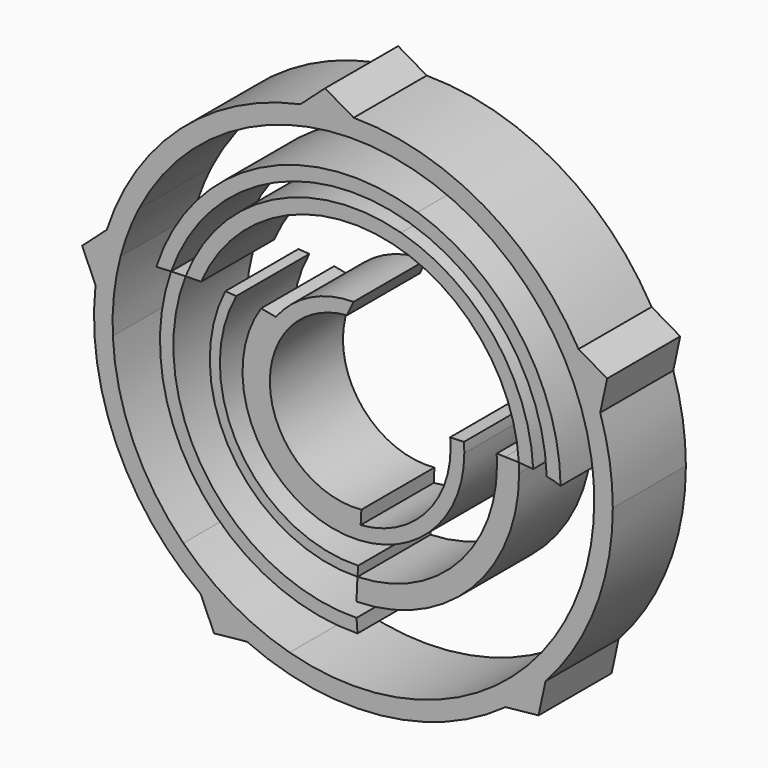
from build123d import *

# Parameters (mm, degrees)
F1_DEPTH = 25.4


with BuildPart() as f1:
    # F0 (on Front) → F1 (new body)
    with BuildSketch(Plane.XZ):
        with BuildLine():
            Line((0.0804563043, 72.1346472531), (-7.8757622136, 76.7543875159))
            Line((-7.8757622136, 76.7543875159), (-14.7280030271, 70.6151523001))
            ThreePointArc((-14.7280030271, 70.6151523001), (-7.3630749336, 71.7579189711), (0.0804563043, 72.1346472531))
        make_face()
        with BuildLine():
            ThreePointArc((62.6077975156, 35.8284453721), (36.2213937543, 62.3812827861), (0.0804563043, 72.1346472531))
            Line((0.0804563043, 72.1346472531), (10.379058307, 66.1548132131))
            ThreePointArc((10.379058307, 66.1548132131), (33.6250311343, 57.9097698478), (52.3091955129, 41.808279412))
            Line((52.3091955129, 41.808279412), (62.6077975156, 35.8284453721))
        make_face()
        with BuildLine():
            Line((10.379058307, 66.1548132131), (0.0804563043, 72.1346472531))
            ThreePointArc((0.0804563043, 72.1346472531), (-7.3630749336, 71.7579189711), (-14.7280030271, 70.6151523001))
            Line((-14.7280030271, 70.6151523001), (-23.5976061943, 62.6684700986))
            ThreePointArc((-23.5976061943, 62.6684700986), (-6.8352870562, 66.6142853558), (10.379058307, 66.1548132131))
        make_face()
        with BuildLine():
            Line((-23.5976061943, 62.6684700986), (-14.7280030271, 70.6151523001))
            ThreePointArc((-14.7280030271, 70.6151523001), (-48.1350992585, 53.7254690711), (-68.5792639553, 22.3673503769))
            Line((-68.5792639553, 22.3673503769), (-59.7096607881, 30.3140325785))
            ThreePointArc((-59.7096607881, 30.3140325785), (-44.684757914, 49.8744079942), (-23.5976061943, 62.6684700986))
        make_face()
        with BuildLine():
            ThreePointArc((68.628988686, 22.214313392), (65.9705211479, 29.1771168386), (62.6077975156, 35.8284453721))
            Line((62.6077975156, 35.8284453721), (52.3091955129, 41.808279412))
            ThreePointArc((52.3091955129, 41.808279412), (61.2417303042, 27.0856905386), (66.1242715931, 10.5718905067))
            Line((66.1242715931, 10.5718905067), (68.628988686, 22.214313392))
        make_face()
        with BuildLine():
            Line((70.5640160335, 31.2087051093), (62.6077975156, 35.8284453721))
            ThreePointArc((62.6077975156, 35.8284453721), (65.9705211479, 29.1771168386), (68.628988686, 22.214313392))
            Line((68.628988686, 22.214313392), (70.5640160335, 31.2087051093))
        make_face()
        with BuildLine():
            ThreePointArc((-70.1811130337, 16.6740871082), (-69.4385618169, 19.5371425839), (-68.5792639553, 22.3673503769))
            Line((-68.5792639553, 22.3673503769), (-75.4315047689, 16.2281151612))
            add(Edge.make_bspline(
                [(-75.4315047689, 16.2281151612), (-73.6801810781, 16.3779407802), (-71.9288512089, 16.5277670762), (-70.1811130337, 16.6740871082)],
                knots=[0, 0, 0, 0, 0.0110848613, 0.0110848613, 0.0110848613, 0.0110848613], degree=3))
        make_face()
        with BuildLine():
            Line((-59.7096607881, 30.3140325785), (-68.5792639553, 22.3673503769))
            ThreePointArc((-68.5792639553, 22.3673503769), (-69.4385618169, 19.5371425839), (-70.1811130337, 16.6740871082))
            add(Edge.make_bspline(
                [(-70.1811130337, 16.6740871082), (-68.362095804, 16.8263745979), (-66.5469692067, 16.9748639956), (-64.7397895139, 17.1156015464)],
                knots=[0.0110848613, 0.0110848613, 0.0110848613, 0.0110848613, 0.0226218032, 0.0226218032, 0.0226218032, 0.0226218032], degree=3))
            ThreePointArc((-64.7397895139, 17.1156015464), (-62.5736850885, 23.8478111585), (-59.7096607881, 30.3140325785))
        make_face()
        with BuildLine():
            ThreePointArc((72.134692122, 0), (71.2528763526, 11.2446173352), (68.628988686, 22.214313392))
            Line((68.628988686, 22.214313392), (66.1242715931, 10.5718905067))
            ThreePointArc((66.1242715931, 10.5718905067), (66.7537762071, 5.3025960338), (66.9640512708, 0))
            ThreePointArc((66.9640512708, 0), (64.145330939, -19.223961125), (55.9264669455, -36.8295324108))
            Line((55.9264669455, -36.8295324108), (53.4217498526, -48.4719552961))
            ThreePointArc((53.4217498526, -48.4719552961), (67.2940386876, -25.9793411127), (72.134692122, 0))
        make_face()
        with BuildLine():
            add(Edge.make_bspline(
                [(-75.4315047689, 16.2281151612), (-73.6801810781, 16.3779407802), (-71.9288512089, 16.5277670762), (-70.1811130337, 16.6740871082)],
                knots=[0, 0, 0, 0, 0.0110848613, 0.0110848613, 0.0110848613, 0.0110848613], degree=3))
            Line((-75.4315047689, 16.2281151612), (-71.7102039728, 7.8141188702))
            ThreePointArc((-71.7102039728, 7.8141188702), (-71.0838323373, 12.2679496162), (-70.1811130337, 16.6740871082))
        make_face()
        with BuildLine():
            add(Edge.make_bspline(
                [(-70.1811130337, 16.6740871082), (-68.362095804, 16.8263745979), (-66.5469692067, 16.9748639956), (-64.7397895139, 17.1156015464)],
                knots=[0.0110848613, 0.0110848613, 0.0110848613, 0.0110848613, 0.0226218032, 0.0226218032, 0.0226218032, 0.0226218032], degree=3))
            ThreePointArc((-70.1811130337, 16.6740871082), (-71.0838323373, 12.2679496162), (-71.7102039728, 7.8141188702))
            Line((-71.7102039728, 7.8141188702), (-66.8933181941, -3.0770348681))
            ThreePointArc((-66.8933181941, -3.0770348681), (-66.5864430839, 7.1013914157), (-64.7397895139, 17.1156015464))
        make_face()
        with BuildLine():
            Line((-66.8933181941, -3.0770348681), (-71.7102039728, 7.8141188702))
            ThreePointArc((-71.7102039728, 7.8141188702), (-65.9705211479, -29.1771168386), (-42.4647723522, -58.3108644818))
            Line((-42.4647723522, -58.3108644818), (-47.2816581308, -47.4197107436))
            ThreePointArc((-47.2816581308, -47.4197107436), (-61.2417303042, -27.0856905386), (-66.8933181941, -3.0770348681))
        make_face()
        with BuildLine():
            ThreePointArc((42.3345913172, -58.4054465401), (48.1350992585, -53.7254690711), (53.4217498526, -48.4719552961))
            Line((53.4217498526, -48.4719552961), (55.9264669455, -36.8295324108))
            ThreePointArc((55.9264669455, -36.8295324108), (44.684757914, -49.8744079942), (30.4879890188, -59.6210255547))
            Line((30.4879890188, -59.6210255547), (42.3345913172, -58.4054465401))
        make_face()
        with BuildLine():
            Line((51.486722505, -57.4663470135), (53.4217498526, -48.4719552961))
            ThreePointArc((53.4217498526, -48.4719552961), (48.1350992585, -53.7254690711), (42.3345913172, -58.4054465401))
            Line((42.3345913172, -58.4054465401), (51.486722505, -57.4663470135))
        make_face()
        with BuildLine():
            ThreePointArc((-29.5913403683, -65.7857612463), (-36.2213937543, -62.3812827861), (-42.4647723522, -58.3108644818))
            Line((-42.4647723522, -58.3108644818), (-38.7434715561, -66.7248607729))
            Line((-38.7434715561, -66.7248607729), (-29.5913403683, -65.7857612463))
        make_face()
        with BuildLine():
            Line((-47.2816581308, -47.4197107436), (-42.4647723522, -58.3108644818))
            ThreePointArc((-42.4647723522, -58.3108644818), (-36.2213937543, -62.3812827861), (-29.5913403683, -65.7857612463))
            Line((-29.5913403683, -65.7857612463), (-17.7447380699, -64.5701822317))
            ThreePointArc((-17.7447380699, -64.5701822317), (-33.6250311343, -57.9097698478), (-47.2816581308, -47.4197107436))
        make_face()
        with BuildLine():
            ThreePointArc((-29.5913403683, -65.7857612463), (7.3630749336, -71.7579189711), (42.3345913172, -58.4054465401))
            Line((42.3345913172, -58.4054465401), (30.4879890188, -59.6210255547))
            ThreePointArc((30.4879890188, -59.6210255547), (6.8352870562, -66.6142853558), (-17.7447380699, -64.5701822317))
            Line((-17.7447380699, -64.5701822317), (-29.5913403683, -65.7857612463))
        make_face()
    extrude(amount=F1_DEPTH)


with BuildPart() as f1b:
    # F0 (on Front) → F1, piece 2 (new body)
    with BuildSketch(Plane.XZ):
        with BuildLine():
            ThreePointArc((17.8474131482, 54.7811527956), (-26.1415508125, 51.3431999277), (-54.7988191164, 17.7930964463))
            add(Edge.make_bspline(
                [(-54.7988191164, 17.7930964463), (-53.4180734669, 17.8701419739), (-52.0468052053, 17.9379460939), (-50.6869602761, 17.9946120432)],
                knots=[0.0440052643, 0.0440052643, 0.0440052643, 0.0440052643, 0.0530367351, 0.0530367351, 0.0530367351, 0.0530367351], degree=3))
            ThreePointArc((-50.6869602761, 17.9946120432), (-24.2822021716, 47.9932147528), (15.5280586181, 51.4961493722))
            add(Edge.make_bspline(
                [(15.5280586181, 51.4961493722), (16.2953998908, 52.5878890346), (17.0695301608, 53.6834646207), (17.8474131482, 54.7811527956)],
                knots=[0.9806259826, 0.9806259826, 0.9806259826, 0.9806259826, 0.9892751554, 0.9892751554, 0.9892751554, 0.9892751554], degree=3))
        make_face()
        with BuildLine():
            add(Edge.make_bspline(
                [(57.6107607755, 0.7107042783), (56.462742198, 1.1538709295), (55.1691307112, 1.5102558583), (53.7564053874, 1.7952393804)],
                knots=[0.6553417422, 0.6553417422, 0.6553417422, 0.6553417422, 0.6691124751, 0.6691124751, 0.6691124751, 0.6691124751], degree=3))
            ThreePointArc((57.6107607755, 0.7107042783), (46.4153784181, 34.1338176009), (17.8474131482, 54.7811527956))
            add(Edge.make_bspline(
                [(15.5280586181, 51.4961493722), (16.2953998908, 52.5878890346), (17.0695301608, 53.6834646207), (17.8474131482, 54.7811527956)],
                knots=[0.9806259826, 0.9806259826, 0.9806259826, 0.9806259826, 0.9892751554, 0.9892751554, 0.9892751554, 0.9892751554], degree=3))
            ThreePointArc((15.5280586181, 51.4961493722), (42.6336645345, 32.7924481089), (53.7564053874, 1.7952393804))
        make_face()
    extrude(amount=F1_DEPTH)


with BuildPart() as f1c:
    # F0 (on Front) → F1, piece 3 (new body)
    with BuildSketch(Plane.XZ):
        with BuildLine():
            add(Edge.make_bspline(
                [(-50.6869602761, 17.9946120432), (-49.3314822975, 18.0510960178), (-47.9873544002, 18.0965132441), (-46.6565038412, 18.1289851741)],
                knots=[0.0530367351, 0.0530367351, 0.0530367351, 0.0530367351, 0.0620392027, 0.0620392027, 0.0620392027, 0.0620392027], degree=3))
            ThreePointArc((-50.6869602761, 17.9946120432), (-43.604859977, -31.4895250996), (1.141385438, -53.7742619093))
            add(Edge.make_bspline(
                [(0.8706699494, -50.0472915148), (0.9119172038, -51.3735505285), (0.9980162573, -52.6210201223), (1.141385438, -53.7742619093)],
                knots=[0.3429048112, 0.3429048112, 0.3429048112, 0.3429048112, 0.3552562401, 0.3552562401, 0.3552562401, 0.3552562401], degree=3))
            ThreePointArc((0.8706699494, -50.0472915148), (-41.0619875564, -28.6252097293), (-46.6565038412, 18.1289851741))
        make_face()
    extrude(amount=F1_DEPTH)


with BuildPart() as f1d:
    # F0 (on Front) → F1, piece 4 (new body)
    with BuildSketch(Plane.XZ):
        with BuildLine():
            ThreePointArc((13.2700106945, 48.2638194748), (-22.4875863699, 44.7191000959), (-46.6565038412, 18.1289851741))
            add(Edge.make_bspline(
                [(-46.6565038412, 18.1289851741), (-45.202639449, 18.1644585655), (-43.7646203485, 18.1844829268), (-42.3449591404, 18.1866091603)],
                knots=[0.0620392027, 0.0620392027, 0.0620392027, 0.0620392027, 0.0718737908, 0.0718737908, 0.0718737908, 0.0718737908], degree=3))
            ThreePointArc((-42.3449591404, 18.1866091603), (-20.6004330804, 41.2246343132), (10.878347446, 44.782919447))
            add(Edge.make_bspline(
                [(10.878347446, 44.782919447), (11.6616317718, 45.9353294378), (12.4601226636, 47.0963501665), (13.2700106945, 48.2638194748)],
                knots=[0.9627272628, 0.9627272628, 0.9627272628, 0.9627272628, 0.9720558065, 0.9720558065, 0.9720558065, 0.9720558065], degree=3))
        make_face()
        with BuildLine():
            add(Edge.make_bspline(
                [(49.9988649095, 2.3670576439), (48.7257298476, 2.5084241824), (47.3905488256, 2.6123363012), (46.0068497112, 2.6866516352)],
                knots=[0.6805676145, 0.6805676145, 0.6805676145, 0.6805676145, 0.6915762269, 0.6915762269, 0.6915762269, 0.6915762269], degree=3))
            ThreePointArc((49.9988649095, 2.3670576439), (39.0815281391, 31.2749678248), (13.2700106945, 48.2638194748))
            add(Edge.make_bspline(
                [(10.878347446, 44.782919447), (11.6616317718, 45.9353294378), (12.4601226636, 47.0963501665), (13.2700106945, 48.2638194748)],
                knots=[0.9627272628, 0.9627272628, 0.9627272628, 0.9627272628, 0.9720558065, 0.9720558065, 0.9720558065, 0.9720558065], degree=3))
            ThreePointArc((10.878347446, 44.782919447), (35.3836876939, 29.5269870209), (46.0068497112, 2.6866516352))
        make_face()
    extrude(amount=F1_DEPTH)


with BuildPart() as f1e:
    # F0 (on Front) → F1, piece 5 (new body)
    with BuildSketch(Plane.XZ):
        with BuildLine():
            ThreePointArc((46.0852288413, 0), (46.0656298913, 1.3438973451), (46.0068497112, 2.6866516352))
            add(Edge.make_bspline(
                [(46.0068497112, 2.6866516352), (44.7919040289, 2.751903606), (43.5395529627, 2.7943377156), (42.2589539711, 2.8192730553)],
                knots=[0.6915762269, 0.6915762269, 0.6915762269, 0.6915762269, 0.701242249, 0.701242249, 0.701242249, 0.701242249], degree=3))
            ThreePointArc((42.2589539711, 2.8192730553), (42.3294012483, 1.4104188191), (42.3528923604, 0))
            ThreePointArc((42.3528923604, 0), (30.301180763, -29.5906393249), (1.0047866298, -42.3409718254))
            add(Edge.make_bspline(
                [(1.0047866298, -42.3409718254), (0.9399173868, -43.6241751634), (0.8905666488, -44.8724435644), (0.8636859405, -46.0771349364)],
                knots=[0.3210190464, 0.3210190464, 0.3210190464, 0.3210190464, 0.3311984622, 0.3311984622, 0.3311984622, 0.3311984622], degree=3))
            ThreePointArc((0.8636859405, -46.0771349364), (32.8911194821, -32.28037448), (46.0852288413, 0))
        make_face()
        with BuildLine():
            ThreePointArc((42.3528923604, 0), (42.3294012483, 1.4104188191), (42.2589539711, 2.8192730553))
            add(Edge.make_bspline(
                [(42.2589539711, 2.8192730553), (41.4598523848, 2.8348328594), (40.6497515192, 2.8435789292), (39.8308764327, 2.8468036855)],
                knots=[0.701242249, 0.701242249, 0.701242249, 0.701242249, 0.7072739057, 0.7072739057, 0.7072739057, 0.7072739057], degree=3))
            ThreePointArc((39.8308764327, 2.8468036855), (39.9070714907, 1.4243081333), (39.9324806219, 0))
            ThreePointArc((39.9324806219, 0), (28.637325364, -27.8299587605), (1.1416721096, -39.9161570472))
            add(Edge.make_bspline(
                [(1.1416721096, -39.9161570472), (1.0911833961, -40.7364829506), (1.0450027701, -41.5454409513), (1.0047866298, -42.3409718254)],
                knots=[0.3147082465, 0.3147082465, 0.3147082465, 0.3147082465, 0.3210190464, 0.3210190464, 0.3210190464, 0.3210190464], degree=3))
            ThreePointArc((1.0047866298, -42.3409718254), (30.301180763, -29.5906393249), (42.3528923604, 0))
        make_face()
    extrude(amount=F1_DEPTH)


with BuildPart() as f1f:
    # F0 (on Front) → F1, piece 6 (new body)
    with BuildSketch(Plane.XZ):
        with BuildLine():
            add(Edge.make_bspline(
                [(-35.621951687, 18.0465943222), (-34.5850294785, 17.9990600754), (-33.5612567748, 17.9387061923), (-32.5517625301, 17.8644322516)],
                knots=[0.087754174, 0.087754174, 0.087754174, 0.087754174, 0.0952866965, 0.0952866965, 0.0952866965, 0.0952866965], degree=3))
            ThreePointArc((-35.621951687, 18.0465943222), (-33.7215443969, -21.3883251357), (1.1416721096, -39.9161570472))
            add(Edge.make_bspline(
                [(1.326030323, -37.1079078778), (1.26069871, -38.0564191035), (1.1984603116, -38.9934788882), (1.1416721096, -39.9161570472)],
                knots=[0.3076100467, 0.3076100467, 0.3076100467, 0.3076100467, 0.3147082465, 0.3147082465, 0.3147082465, 0.3147082465], degree=3))
            ThreePointArc((1.326030323, -37.1079078778), (-31.6109337539, -19.480863705), (-32.5517625301, 17.8644322516))
        make_face()
    extrude(amount=F1_DEPTH)


with BuildPart() as f1g:
    # F0 (on Front) → F1, piece 7 (new body)
    with BuildSketch(Plane.XZ):
        with BuildLine():
            add(Edge.make_bspline(
                [(-25.6645379323, 17.0925479942), (-24.2548098485, 16.8725866776), (-22.8835176436, 16.6151552991), (-21.5545197047, 16.3164929872)],
                knots=[0.1130457972, 0.1130457972, 0.1130457972, 0.1130457972, 0.1243919933, 0.1243919933, 0.1243919933, 0.1243919933], degree=3))
            ThreePointArc((-25.6645379323, 17.0925479942), (-26.75376959, -15.3316508223), (1.7721063726, -30.7844659401))
            add(Edge.make_bspline(
                [(2.0184674831, -26.9583206473), (1.9430941028, -28.2379532102), (1.8592908583, -29.5154271132), (1.7721063726, -30.7844659401)],
                knots=[0.2830165775, 0.2830165775, 0.2830165775, 0.2830165775, 0.2921665644, 0.2921665644, 0.2921665644, 0.2921665644], degree=3))
            ThreePointArc((2.0184674831, -26.9583206473), (-23.7400865179, -12.9318813491), (-21.5545197047, 16.3164929872))
        make_face()
        with BuildLine():
            ThreePointArc((30.8354293664, 0), (30.8052215855, 1.3645612049), (30.7146574284, 2.726448838))
            add(Edge.make_bspline(
                [(30.7146574284, 2.726448838), (29.4439156689, 2.6969565272), (28.1715468265, 2.6655768286), (26.9049012864, 2.6365791987)],
                knots=[0.7290704359, 0.7290704359, 0.7290704359, 0.7290704359, 0.7380535345, 0.7380535345, 0.7380535345, 0.7380535345], degree=3))
            ThreePointArc((26.9049012864, 2.6365791987), (27.0015411264, 1.3198635918), (27.0337800372, 0))
            ThreePointArc((27.0337800372, 0), (19.8165596037, -18.3882905289), (2.0184674831, -26.9583206473))
            add(Edge.make_bspline(
                [(2.0184674831, -26.9583206473), (1.9430941028, -28.2379532102), (1.8592908583, -29.5154271132), (1.7721063726, -30.7844659401)],
                knots=[0.2830165775, 0.2830165775, 0.2830165775, 0.2830165775, 0.2921665644, 0.2921665644, 0.2921665644, 0.2921665644], degree=3))
            ThreePointArc((1.7721063726, -30.7844659401), (22.4217234517, -21.1681369436), (30.8354293664, 0))
        make_face()
        with BuildLine():
            ThreePointArc((0.0308885054, 27.0337623908), (-12.0221312947, 24.2135008257), (-21.5545197047, 16.3164929872))
            add(Edge.make_bspline(
                [(-21.5545197047, 16.3164929872), (-20.1643054515, 16.0040736894), (-18.8203715182, 15.6465376189), (-17.5271344034, 15.2395798985)],
                knots=[0.1243919933, 0.1243919933, 0.1243919933, 0.1243919933, 0.136260818, 0.136260818, 0.136260818, 0.136260818], degree=3))
            ThreePointArc((-17.5271344034, 15.2395798985), (-10.4381626353, 20.7482528584), (-1.7896155874, 23.1569106732))
            add(Edge.make_bspline(
                [(-1.7896155874, 23.1569106732), (-1.2533807016, 24.4091596989), (-0.6435000896, 25.7031724079), (0.0308885054, 27.0337623908)],
                knots=[0.8993224909, 0.8993224909, 0.8993224909, 0.8993224909, 0.9118099368, 0.9118099368, 0.9118099368, 0.9118099368], degree=3))
        make_face()
        with BuildLine():
            add(Edge.make_bspline(
                [(-21.5545197047, 16.3164929872), (-20.1643054515, 16.0040736894), (-18.8203715182, 15.6465376189), (-17.5271344034, 15.2395798985)],
                knots=[0.1243919933, 0.1243919933, 0.1243919933, 0.1243919933, 0.136260818, 0.136260818, 0.136260818, 0.136260818], degree=3))
            ThreePointArc((-21.5545197047, 16.3164929872), (-23.7400865179, -12.9318813491), (2.0184674831, -26.9583206473))
            add(Edge.make_bspline(
                [(2.214209568, -23.120175429), (2.1607511248, -24.3975335956), (2.0938221425, -25.6790059153), (2.0184674831, -26.9583206473)],
                knots=[0.2738688632, 0.2738688632, 0.2738688632, 0.2738688632, 0.2830165775, 0.2830165775, 0.2830165775, 0.2830165775], degree=3))
            ThreePointArc((2.214209568, -23.120175429), (-20.6516131077, -10.628081291), (-17.5271344034, 15.2395798985))
        make_face()
    extrude(amount=F1_DEPTH)


solid = Compound([f1.part, f1b.part, f1c.part, f1d.part, f1e.part, f1f.part, f1g.part])
